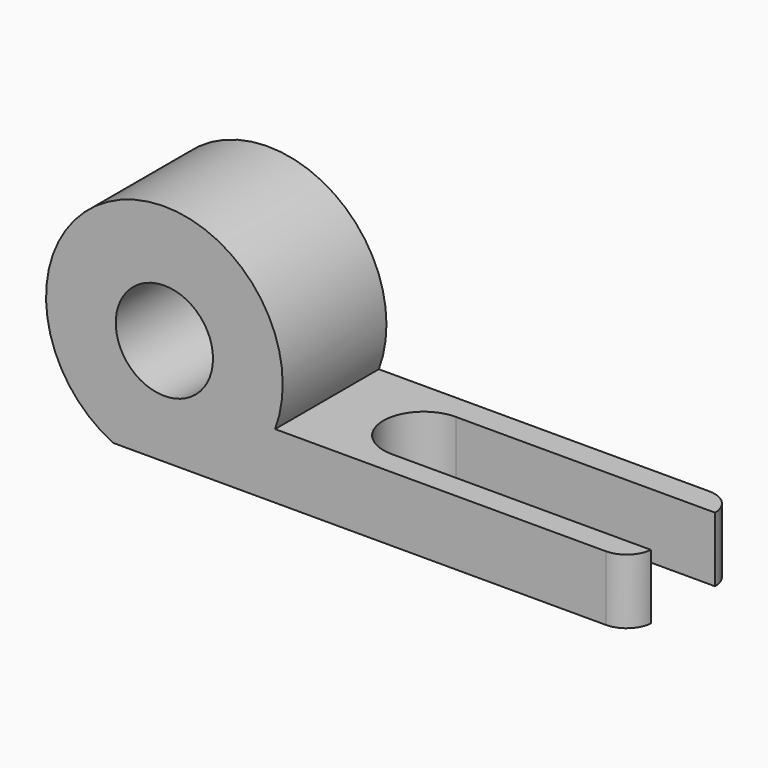
from build123d import *

# Parameters (mm, degrees)
F0_R        = 9.525
F2_DEPTH    = 25.4
F3_W        = 50.8
F3_H        = 15.748
F4_DEPTH    = 25.4
F5_T1_DEPTH = 38.0949194415
F5_T3_DEPTH = 38.0185897363


# Not quite as in the source:
# - a fillet or chamfer that OpenCascade refuses, or shapes differently, is made with other operations: its cross-section is extruded or revolved along the edge and cut away or added


with BuildPart() as f2:
    # F0 (on Front) → F2 (new body)
    with BuildSketch(Plane.XZ):
        with BuildLine():
            ThreePointArc((-20.9804001153, 12.7), (-51.2752635033, 42.3996584702), (-52.7304001153, 0))
            Line((-52.7304001153, 0), (48.8695998847, 0))
            Line((48.8695998847, 0), (48.8695998847, 12.7))
            Line((48.8695998847, 12.7), (-20.9804001153, 12.7))
        make_face()
        with Locations((-42.6671736259, 20.8794337765)):
            Circle(F0_R, mode=Mode.SUBTRACT)
    extrude(amount=F2_DEPTH)

    # F3 (on face) → F4 (cut)
    with BuildSketch(Plane.XY.offset(12.7)):
        with Locations((23.4695998847, -12.8523994962)):
            Rectangle(F3_W, F3_H)
        with BuildLine():
            ThreePointArc((-1.9304001153, -4.9783994962), (-9.8044001153, -12.8523994962), (-1.9304001153, -20.7263994962))
            Line((-1.9304001153, -20.7263994962), (-1.9304001153, -4.9783994962))
        make_face()
    extrude(amount=-F4_DEPTH, mode=Mode.SUBTRACT)

    # F5: fillet of radius 5.08 on 2 edges, made by hand

    # F5_s2 → F5_t1 (cut)
    with BuildSketch(Plane.XY.offset(-12.6974597208)):
        with BuildLine():
            ThreePointArc((43.7906159964, 0), (47.3466158165, -1.4521541819), (48.8695998847, -4.9783994962))
            Line((48.8695998847, -4.9783994962), (48.8695998847, 0))
            Line((48.8695998847, 0), (43.7906159964, 0))
        make_face()
    extrude(amount=F5_T1_DEPTH, mode=Mode.SUBTRACT)

    # F5_s4 → F5_t3 (cut)
    with BuildSketch(Plane.XY.offset(-12.6592948682)):
        with BuildLine():
            ThreePointArc((48.8695998847, -20.7263994962), (47.2513057546, -24.0530221966), (43.8058819375, -25.4))
            Line((43.8058819375, -25.4), (48.8695998847, -25.4))
            Line((48.8695998847, -25.4), (48.8695998847, -20.7263994962))
        make_face()
    extrude(amount=F5_T3_DEPTH, mode=Mode.SUBTRACT)


solid = f2.part
